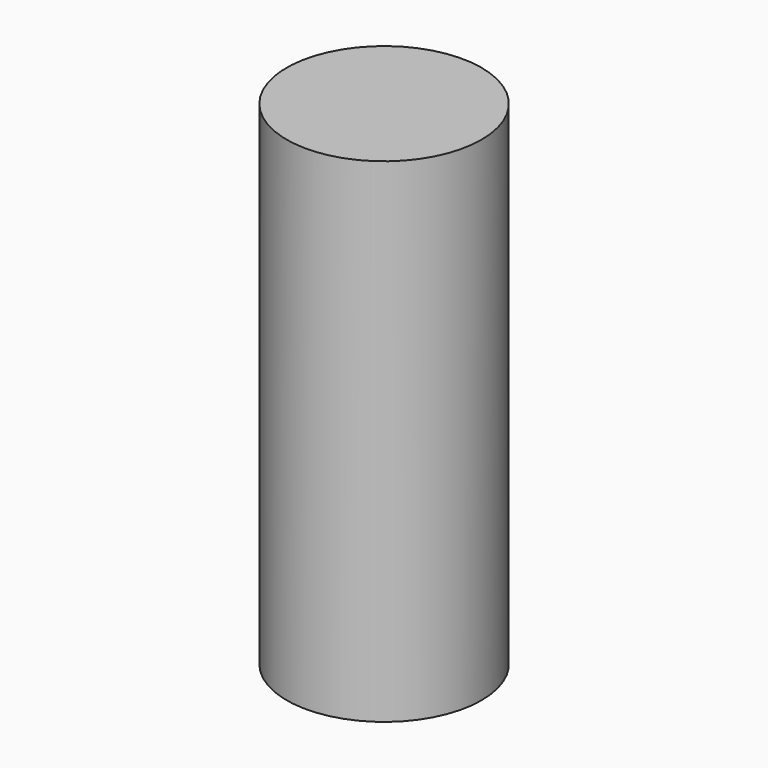
from build123d import *

# Parameters (mm, degrees)
F3_R     = 16.3715148317
F4_DEPTH = 82.92141


# Not quite as in the source:
# - a feature of the source that left no trace in its solid (it failed there, or was rolled back) is left out
# - the program builds the solid bodies; features that only make, move or delete a surface that nothing else refers to are left out


with BuildPart() as f4:
    # F3 (on face) → F4 (new body)
    with BuildSketch(Plane(origin=(0, 0, -35.9900146723), x_dir=(1, 0, 0), z_dir=(0, 0, -1))):
        with Locations((5.0615929067, 0)):
            Circle(F3_R)
    extrude(amount=-F4_DEPTH)


solid = f4.part
